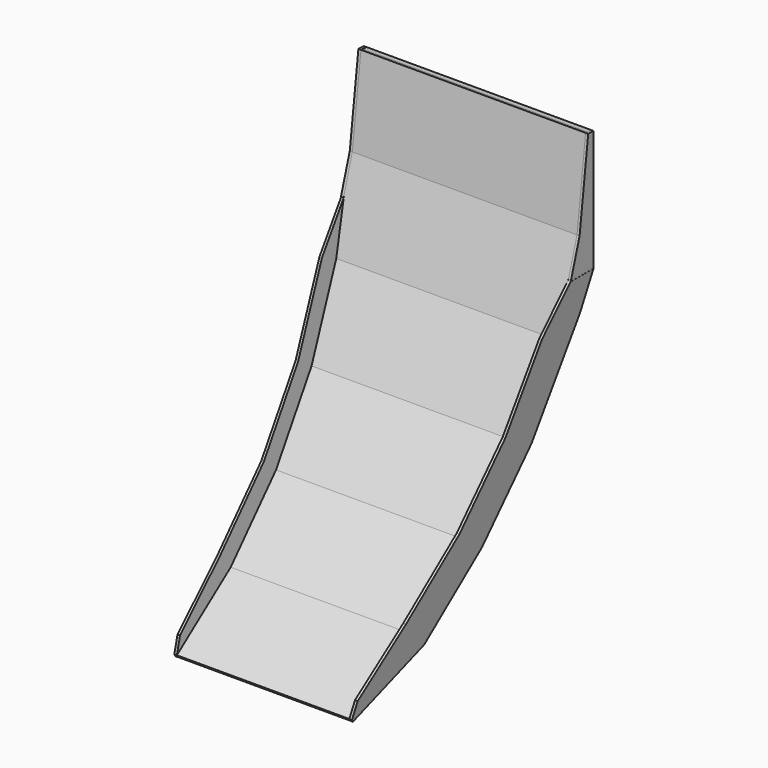
from build123d import *

# Parameters (mm, degrees)
F0_W      = 260
F0_H      = 140
F1_DEPTH  = 5
F3_DEPTH  = 130
F7_W      = 657.2483032942
F7_H      = 632.9057961702
F8_DEPTH  = 174
F12_DEPTH = 3
F14_DEPTH = 3
F16_DEPTH = 1.5


with BuildPart() as f1:
    # F0 (on Front) → F1 (new body)
    with BuildSketch(Plane.XZ):
        Rectangle(F0_W, F0_H)
    extrude(amount=F1_DEPTH)


with BuildPart() as f3:
    # F2 (on Right) → F3 (new body, symmetric)
    with BuildSketch(Plane.YZ):
        Polygon((-17.4873212862, -29.2172707098), (-5, 70), (-7.9765181213, 70.3746196386), (-20.4310644359, -28.5822394788), (-49.8025794157, -123.622248239), (-95.2313994122, -212.1180756609), (-155.3371927178, -291.3808208093), (-228.2936752181, -359.0021252816), (-312.1046553088, -413.0696322199), (-310.4783616328, -415.5905782486), (-226.4468273432, -361.3807890501), (-153.1053519834, -293.4026455624), (-92.6823791695, -213.7216292766), (-47.013830355, -124.7588075522), align=None)
    extrude(amount=F3_DEPTH, both=True)


with BuildPart() as f8:
    # F7 (on face) → F8 (new body)
    with BuildSketch(Plane(origin=(134.8891541046, 0, -11.8012718167), x_dir=(0, -1, 0), z_dir=(-0.9961946981, 0, 0.0871557427))):
        with Locations((150.0718072057, -147.6648971438)):
            Rectangle(F7_W, F7_H)
    extrude(amount=-F8_DEPTH)


with BuildPart() as f9_1:
    # F9: instance of F8
    add(f8.part.mirror(Plane.YZ))


with BuildPart() as f3_1:
    add(f3.part)

    # F10: cut F9_1, F8
    add(f9_1.part, mode=Mode.SUBTRACT)
    add(f8.part, mode=Mode.SUBTRACT)


with BuildPart() as f12:
    # F11 (on face) → F12 (new body)
    with BuildSketch(Plane(origin=(134.8891541046, 0, -11.8012718167), x_dir=(0, -1, 0), z_dir=(-0.9961946981, 0, 0.0871557427))):
        Polygon((305.6514709987, -385.5638570208), (241.8128323534, -331.6166724948), (171.4191538735, -266.1215299442), (113.4206222217, -189.3455181509), (69.5816849654, -103.6205900856), (33.2255263913, -58.4033823092), (0, -58.4033823092), (15.1668360589, -98.9159475502), (73.139217219, -212.2781437109), (135.6694516868, -295.0530326988), (211.573731067, -365.6753059705), (310.4783616328, -405.3317159841), (312.1046553088, -402.8011403512), align=None)
    extrude(amount=-F12_DEPTH)


with BuildPart() as f14:
    # F13 (on face) → F14 (new body)
    with BuildSketch(Plane.YZ.offset(130)):
        Polygon((0, 70), (-7.9765181213, 70.3746196386), (-20.4310644359, -28.5822394788), (-33.230961968, -70), (0, -70), align=None)
    extrude(amount=F14_DEPTH)


with BuildPart() as f16:
    # F15 (on Right) → F16 (new body, symmetric)
    with BuildSketch(Plane.YZ):
        Polygon((-30.0909664235, -70), (-5, -70), (-5, 70), (-17.4873212862, -29.2172707098), (-29.3753939774, -67.684558948), align=None)
    extrude(amount=F16_DEPTH, both=True)


with BuildPart() as f17_1:
    # F17: instance of F14
    add(f14.part.mirror(Plane.YZ))


with BuildPart() as f17_2:
    # F17: instance of F12
    add(f12.part.mirror(Plane.YZ))


solid = Compound([f1.part, f3_1.part, f12.part, f14.part, f16.part, f17_1.part, f17_2.part])
